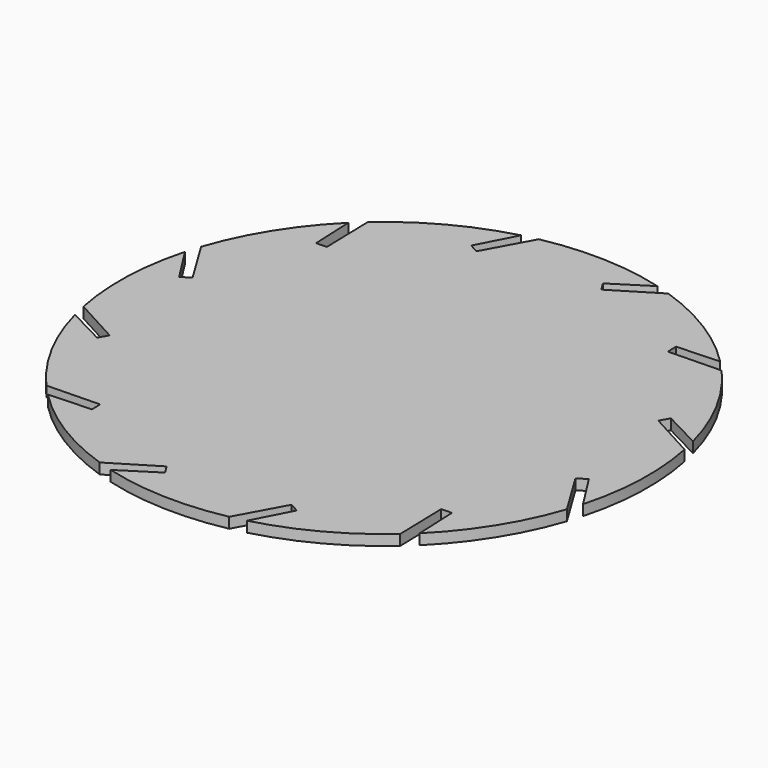
from build123d import *

# Parameters (mm, degrees)
F0_R            = 75
F1_DEPTH        = 3
F3_DEPTH        = 3
F3_COPIES_COUNT = 12


# Not quite as in the source:
# - a pattern or mirror of a feature is missing from the dataset's text; its kind, count and spacing are read off the source's solid


with BuildPart() as f1:
    # F0 (on Top) → F1 (new body)
    with BuildSketch(Plane.XY):
        Circle(F0_R)
    extrude(amount=F1_DEPTH)

    # F2 (on Top) → F3 (cut, through all)
    with BuildSketch(Plane.XY):
        with BuildLine():
            Line((23.905803232, 71.0880620909), (28.1729654475, 73.6940794788))
            Line((28.1729654475, 73.6940794788), (19.7568770352, 72.3509903859))
            ThreePointArc((19.7568770352, 72.3509903859), (21.840470668, 71.7495215385), (23.905803232, 71.0880620909))
        make_face()
        with BuildLine():
            Line((11.1043165854, 63.2700099269), (23.905803232, 71.0880620909))
            ThreePointArc((23.905803232, 71.0880620909), (21.840470668, 71.7495215385), (19.7568770352, 72.3509903859))
            Line((19.7568770352, 72.3509903859), (9.5407061526, 65.8303072562))
            Line((9.5407061526, 65.8303072562), (11.1043165854, 63.2700099269))
        make_face()
    f3 = extrude(amount=F3_DEPTH, mode=Mode.SUBTRACT)

    # F3_copies: F3 ×12 about axis
    f3_copies_axis = Axis((0, 0, 0), (0, 0, 1))
    for i in range(1, F3_COPIES_COUNT):
        add(f3.rotate(f3_copies_axis, i * 360 / F3_COPIES_COUNT), mode=Mode.SUBTRACT)


solid = f1.part
